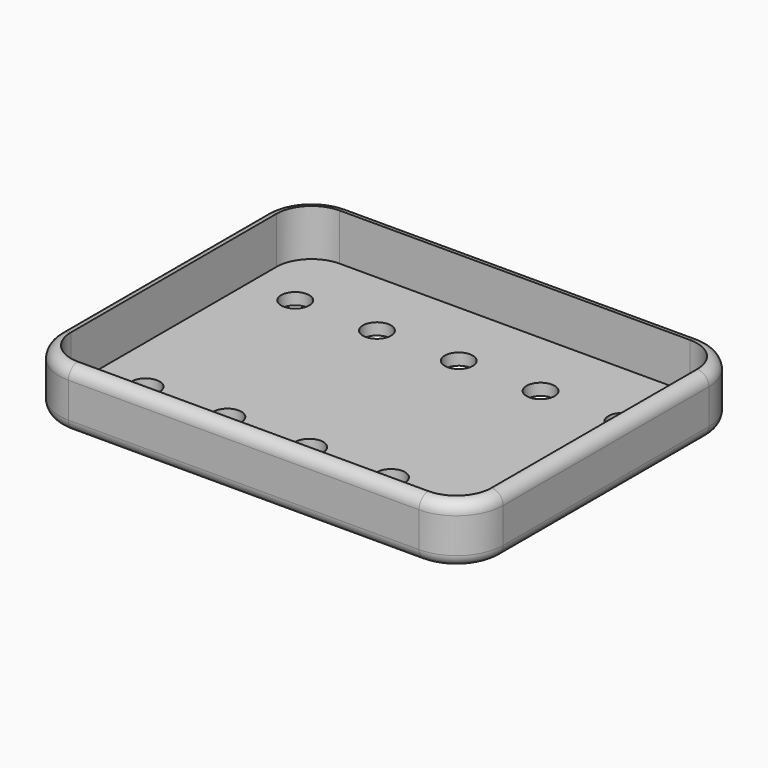
from build123d import *

# Parameters (mm, degrees)
F2_DEPTH = 3.175
F3_R     = 1.27
F4_T     = -1.27
F1_R     = 1.524
F5_DEPTH = 25.4


# Not quite as in the source:
# - a shell that OpenCascade refuses in one call is made with other operations: the cavity is built on its own and cut out


with BuildPart() as f2:
    # F0 (on Top) → F2 (new body, symmetric)
    with BuildSketch(Plane.XY):
        with BuildLine():
            ThreePointArc((24.13, 13.97), (22.6421024484, 17.5621024484), (19.05, 19.05))
            Line((19.05, 19.05), (-19.05, 19.05))
            ThreePointArc((-19.05, 19.05), (-22.6421024484, 17.5621024484), (-24.13, 13.97))
            Line((-24.13, 13.97), (-24.13, -13.97))
            ThreePointArc((-24.13, -13.97), (-22.6421024484, -17.5621024484), (-19.05, -19.05))
            Line((-19.05, -19.05), (19.05, -19.05))
            ThreePointArc((19.05, -19.05), (22.6421024484, -17.5621024484), (24.13, -13.97))
            Line((24.13, -13.97), (24.13, 13.97))
        make_face()
    extrude(amount=F2_DEPTH, both=True)

    # F3
    f3_edges = [f2.edges().sort_by_distance(p)[0] for p in [
        (-24.13, 0, 3.175),
        (-24.13, 0, -3.175),
    ]]
    fillet(f3_edges, radius=F3_R)

    # F4: a shell. OpenCascade refuses it in one call, so the cavity is built on its own and cut out:
    # the body offset inwards by the wall thickness, plus a prism from it out through each open face.
    f4_core = offset(f2.part, amount=F4_T, kind=Kind.INTERSECTION, mode=Mode.PRIVATE)
    f4_exits = [f4_core.faces().sort_by_distance(p)[0] for p in [
        (0, 0, 1.905),
    ]]
    add(f4_core, mode=Mode.SUBTRACT)
    extrude(f4_exits, amount=-F4_T, mode=Mode.SUBTRACT)

    # F1 (on Top) → F5 (cut)
    with BuildSketch(Plane.XY):
        with Locations((-17.78, 10.16)):
            Circle(F1_R)
        with Locations((-17.78, -10.16)):
            Circle(F1_R)
        with Locations((-8.89, 10.16)):
            Circle(F1_R)
        with Locations((0, 10.16)):
            Circle(F1_R)
        with Locations((8.89, 10.16)):
            Circle(F1_R)
        with Locations((17.78, 10.16)):
            Circle(F1_R)
        with Locations((-8.89, -10.16)):
            Circle(F1_R)
        with Locations((0, -10.16)):
            Circle(F1_R)
        with Locations((8.89, -10.16)):
            Circle(F1_R)
        with Locations((17.78, -10.16)):
            Circle(F1_R)
    extrude(amount=-F5_DEPTH, mode=Mode.SUBTRACT)


solid = f2.part
